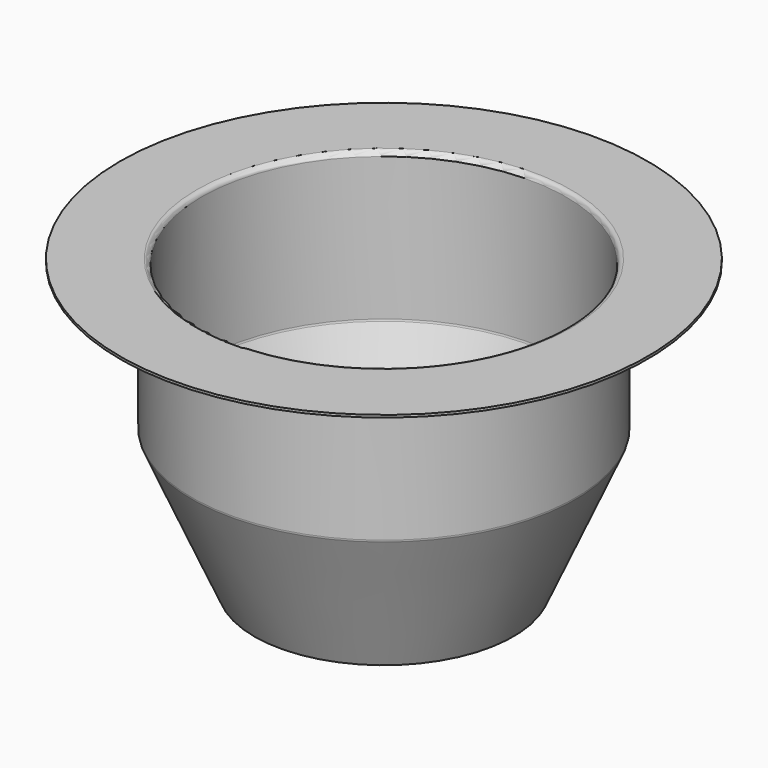
from build123d import *


# Not quite as in the source:
# - a feature names something its author has since deleted; it is built from what else it names


with BuildPart() as f1:
    # F0 (on Front) → F1 (revolve)
    with BuildSketch(Plane.XZ):
        with BuildLine():
            Line((-55, 60), (-41, 60))
            ThreePointArc((-41, 60), (-40.2928932188, 59.7071067812), (-40, 59))
            Line((-40, 59), (-40, 29.71056928))
            ThreePointArc((-40, 29.71056928), (-39.9785413088, 29.5045185412), (-39.9150861861, 29.3073109607))
            Line((-39.9150861861, 29.3073109607), (-27, 0))
            Line((-27, 0), (-25, 0))
            Line((-25, 0), (-37.9150861861, 29.3073109607))
            ThreePointArc((-37.9150861861, 29.3073109607), (-37.9785413088, 29.5045185412), (-38, 29.71056928))
            Line((-38, 29.71056928), (-38, 59.5))
            ThreePointArc((-38, 59.5), (-38.2928932188, 60.2071067812), (-39, 60.5))
            Line((-39, 60.5), (-55, 60.5))
            Line((-55, 60.5), (-55, 60))
        make_face()
    revolve(axis=Axis((0, 0, 19.5262523685), (0, 0, 1)))


solid = f1.part
